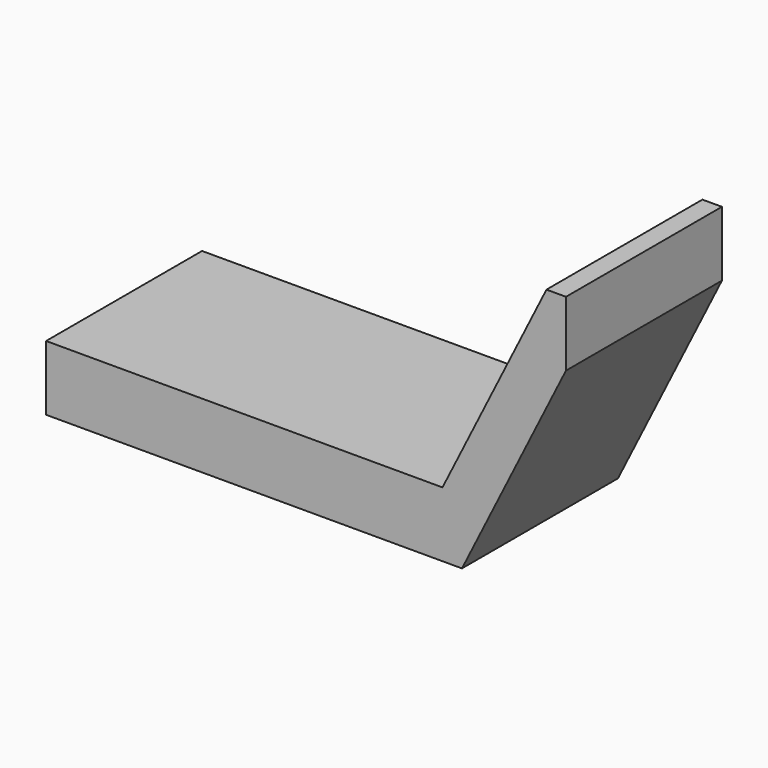
from build123d import *

# Parameters (mm, degrees)
F0_W     = 50.8
F0_H     = 6.35
F1_DEPTH = 19.05
F2_W     = 12.065
F2_H     = 19.05
F3_DEPTH = 20.32
F4_SIZE2 = 10.16
F4_SIZE  = 20.32
F5_SIZE2 = 20.31999
F5_SIZE  = 10.15999


# Not quite as in the source:
# - a fillet or chamfer is up to 0.001 mm smaller than in the source, because OpenCascade refuses the exact size


with BuildPart() as f1:
    # F0 (on Front) → F1 (new body)
    with BuildSketch(Plane.XZ):
        with Locations((25.4, -3.175)):
            Rectangle(F0_W, F0_H)
    extrude(amount=F1_DEPTH)

    # F2 (on face) → F3 (join)
    with BuildSketch(Plane.XY):
        with Locations((44.7675, -9.525)):
            Rectangle(F2_W, F2_H)
    extrude(amount=F3_DEPTH)

    # F4
    f4_edges = [f1.edges().sort_by_distance(p)[0] for p in [
        (50.8, -9.525, -6.35),
    ]]
    f4_side = f1.faces().sort_by_distance((50.8, -9.525, 6.985))[0]
    chamfer(f4_edges, length=F4_SIZE, length2=F4_SIZE2, reference=f4_side)

    # F5 (size 10.16 and 20.32 in the source; OpenCascade refuses exactly that, so slightly less here)
    f5_edges = [f1.edges().sort_by_distance(p)[0] for p in [
        (38.735, -9.525, 20.32),
    ]]
    f5_side = f1.faces().sort_by_distance((44.7675, -9.525, 20.32))[0]
    chamfer(f5_edges, length=F5_SIZE, length2=F5_SIZE2, reference=f5_side)


solid = f1.part
